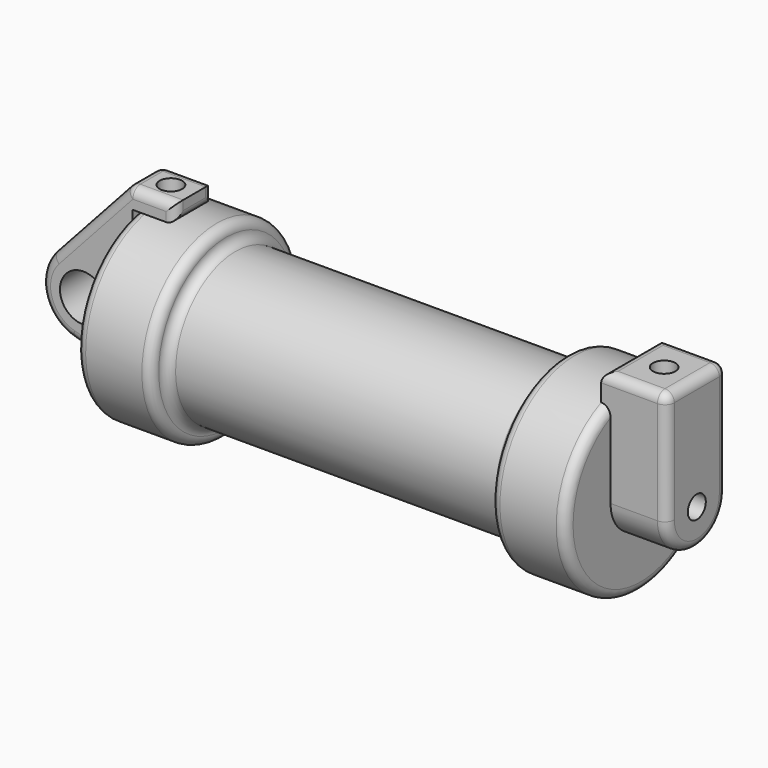
from build123d import *

# Parameters (mm, degrees)
F0_W      = 5.842
F0_H      = 12.7
F0_R      = 3.175
F2_DEPTH  = 3.175
F4_DEPTH  = 1.27
F5_DEPTH  = 7.62
F6_DEPTH  = 66.294
F8_R      = 1.524
F9_DEPTH  = 10.414
F10_R     = 1.524
F11_DEPTH = 17.78
F12_R     = 1.27
F12_2_R   = 1.27
F13_R     = 1.26999


# Not quite as in the source:
# - a fillet or chamfer is up to 0.001 mm smaller than in the source, because OpenCascade refuses the exact size


with BuildPart() as f1:
    # F0 (on Front) → F1 (revolve)
    with BuildSketch(Plane.XZ):
        with Locations((2.921, 6.35)):
            Rectangle(F0_W, F0_H)
        Polygon((5.842, 12.7), (5.842, 0), (66.294, 0), (66.294, 12.7), (56.134, 12.7), (56.134, 10.16), (10.16, 10.16), (10.16, 12.7), align=None)
    revolve(axis=Axis((33.147, 0, 0), (-1, 0, 0)))

    # F3 (on face) → F4 (join)
    with BuildSketch(Plane.YZ.offset(66.294)):
        with BuildLine():
            Line((-5.08, 15.24), (-5.08, 11.6397422652))
            ThreePointArc((-5.08, 11.6397422652), (0, 12.7), (5.08, 11.6397422652))
            Line((5.08, 11.6397422652), (5.08, 15.24))
            Line((5.08, 15.24), (-5.08, 15.24))
        make_face()
    extrude(amount=-F4_DEPTH)

    # F3 (on face) → F5 (join)
    with BuildSketch(Plane.YZ.offset(66.294)):
        with BuildLine():
            ThreePointArc((5.08, 0), (0, 5.08), (-5.08, 0))
            ThreePointArc((-5.08, 0), (0, -5.08), (5.08, 0))
        make_face()
        with BuildLine():
            ThreePointArc((-1.524, 0), (0, 1.524), (1.524, 0))
            ThreePointArc((1.524, 0), (0, -1.524), (-1.524, 0))
        make_face(mode=Mode.SUBTRACT)
        with BuildLine():
            Line((-5.08, 15.24), (-5.08, 0))
            ThreePointArc((-5.08, 0), (0, 5.08), (5.08, 0))
            Line((5.08, 0), (5.08, 15.24))
            Line((5.08, 15.24), (-5.08, 15.24))
        make_face()
    extrude(amount=F5_DEPTH)

    # F6 (cut, through all): a face of the model
    f6_faces = [f1.faces().sort_by_distance(p)[0] for p in [
        (66.294, 0, 0),
    ]]
    extrude(f6_faces, amount=-F6_DEPTH, mode=Mode.SUBTRACT)

    # F8 (on face) → F9 (cut)
    with BuildSketch(Plane.XY.offset(15.24)):
        with Locations((69.501914084, -0.015315949)):
            Circle(F8_R)
    extrude(amount=-F9_DEPTH, mode=Mode.SUBTRACT)

    # F12
    f12_edges = [f1.edges().sort_by_distance(p)[0] for p in [
        (0, 0, -12.7),
        (10.16, 0, -12.7),
    ]]
    fillet(f12_edges, radius=F12_R)

    # F13 (radius 1.27 in the source; OpenCascade refuses exactly that, so slightly less here)
    f13_edges = [f1.edges().sort_by_distance(p)[0] for p in [
        (66.294, 0, -12.7),
        (56.134, 0, -12.7),
        (73.914, 0, 15.24),
        (73.914, -5.08, 7.62),
        (70.104, -5.08, 0),
        (69.469, -5.08, 15.24),
        (65.024, 0, 15.24),
        (69.469, 5.08, 15.24),
        (56.134, 0, -10.16),
        (10.16, 0, -10.16),
        (33.147, 0, 10.16),
        (73.914, 0, -5.08),
        (73.914, 5.08, 7.62),
    ]]
    fillet(f13_edges, radius=F13_R)


with BuildPart() as f2:
    # F0 (on Front) → F2 (new body, symmetric)
    with BuildSketch(Plane.XZ):
        with BuildLine():
            Line((5.842, 0), (0, 0))
            Line((0, 0), (-0.9398, 0))
            ThreePointArc((-0.9398, 0), (-3.1957909266, -4.5493385486), (-8.1826630726, -5.5069827884))
            Line((-8.1826630726, -5.5069827884), (5.842, -9.398))
            Line((5.842, -9.398), (5.842, 0))
        make_face()
        with BuildLine():
            ThreePointArc((-8.1826630726, -5.5069827884), (-3.1957909266, -4.5493385486), (-0.9398, 0))
            ThreePointArc((-0.9398, 0), (-4.5919612295, 5.3297205562), (-10.8806298187, 3.8475430269))
            ThreePointArc((-10.8806298187, 3.8475430269), (-12.1459778134, -1.5837270034), (-8.1826630726, -5.5069827884))
        make_face()
        with Locations((-6.6548, 0)):
            Circle(F0_R, mode=Mode.SUBTRACT)
        with BuildLine():
            Line((-0.9398, 0), (0, 0))
            Line((0, 0), (0, 12.7))
            Line((0, 12.7), (5.842, 12.7))
            Line((5.842, 12.7), (5.842, 15.24))
            Line((5.842, 15.24), (-0.508, 15.24))
            Line((-0.508, 15.24), (-10.8806298187, 3.8475430269))
            ThreePointArc((-10.8806298187, 3.8475430269), (-4.5919612295, 5.3297205562), (-0.9398, 0))
        make_face()
    extrude(amount=F2_DEPTH, both=True)

    # F10 (on face) → F11 (cut)
    with BuildSketch(Plane.XY.offset(15.24)):
        with Locations((2.667, 0)):
            Circle(F10_R)
    extrude(amount=-F11_DEPTH, mode=Mode.SUBTRACT)

    # F12#2
    f12_2_edges = [f2.edges().sort_by_distance(p)[0] for p in [
        (-5.694315, -3.175, 9.543772),
        (-5.694315, 3.175, 9.543772),
        (-10.88063, 0, 3.847543),
        (-0.508, 0, 15.24),
        (2.667, -3.175, 15.24),
        (2.667, 3.175, 15.24),
        (5.842, 0, 12.7),
        (5.842, -3.175, 13.97),
        (5.842, 3.175, 13.97),
        (-8.182663, 0, -5.506983),
        (-1.170332, -3.175, -7.452491),
        (-1.170332, 3.175, -7.452491),
        (-12.145978, 3.175, -1.583727),
        (-12.145978, -3.175, -1.583727),
    ]]
    fillet(f12_2_edges, radius=F12_2_R)


solid = Compound([f1.part, f2.part])
